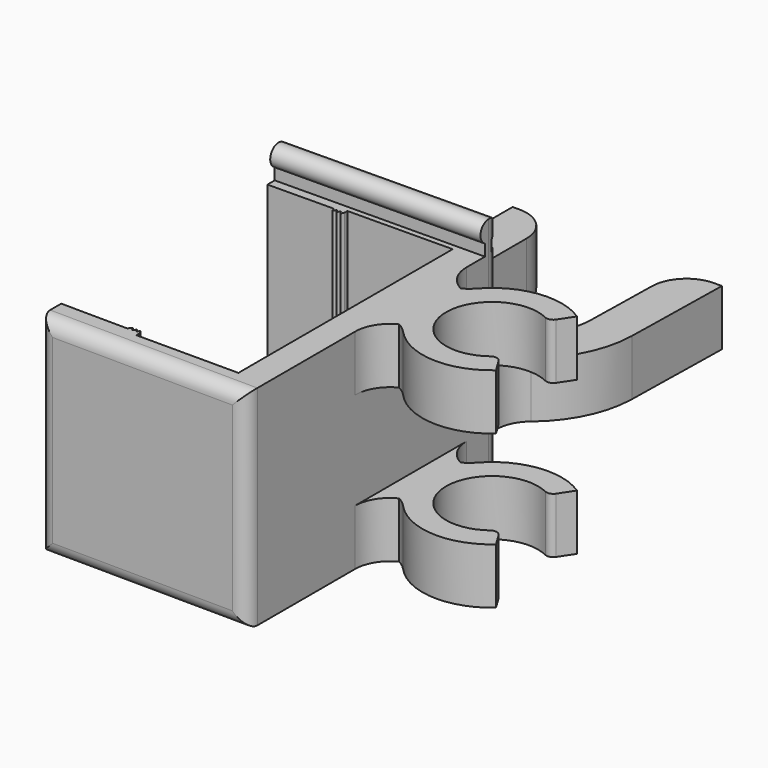
from build123d import *

# Parameters (mm, degrees)
F1_DEPTH     = 30
F2_DEPTH     = 8
F5_DEPTH     = 8
F6_W         = 15
F6_H         = 8
F7_DEPTH     = 17
F10_DEPTH    = 8
F12_REACH    = 53.956775782
F13_T1_DEPTH = 8
F13_T3_DEPTH = 8
F13_T5_DEPTH = 33
F13_T7_DEPTH = 32.520696372
F14_R        = 2
F15_R        = 1


# Not quite as in the source:
# - a fillet or chamfer that OpenCascade refuses, or shapes differently, is made with other operations: its cross-section is extruded or revolved along the edge and cut away or added


with BuildPart() as f1:
    # F0 (on Top) → F1 (new body)
    with BuildSketch(Plane.XY):
        Polygon((-19.4335049985, 21.8533294287), (-19.3985988565, 17.8534817365), (-9.9558601587, 17.9358872687), (-9.7491024062, 17.4549428523), (-9.4364569921, 17.9404200315), (-9.1781169176, 17.4304714203), (-8.9225616318, 17.9449047283), (-8.6024082196, 17.4476796256), (-8.3908626536, 17.949544795), (-8.3952257552, 18.4495067188), (6.6091373464, 18.5804478119), (6.6091373464, 18.0804478119), (6.6091373464, -19.3734843389), (6.6259289407, -19.8732023017), (-8.0640320303, -19.8732023017), (-8.0233838527, -19.2457882609), (-8.3196364677, -18.7431838643), (-8.5862603211, -19.2408761124), (-8.8343713433, -18.7508519739), (-9.1803468433, -19.2356915979), (-9.4099212438, -18.7637861818), (-9.9014025182, -19.2293990403), (-19.3985988565, -19.1465182635), (-19.3985988565, -23.1465182635), (10.5653526934, -23.4080097072), (10.5653526934, 1.1284245411), (10.5653526934, 11.1284245411), (10.5653526934, 22.1151254937), align=None)
    extrude(amount=F1_DEPTH)

    # F0 (on Top) → F2 (join)
    with BuildSketch(Plane.XY):
        with BuildLine():
            Line((13.4887376895, 11.1284245411), (10.5653526934, 11.1284245411))
            Line((10.5653526934, 11.1284245411), (10.5653526934, 1.1284245411))
            Line((10.5653526934, 1.1284245411), (13.558922693, 1.1284245411))
            ThreePointArc((13.558922693, 1.1284245411), (20.5784668777, -3.6810997137), (28.7603608072, -1.3439784408))
            Line((28.7603608072, -1.3439784408), (27.5756506747, 0.610225606))
            ThreePointArc((27.5756506747, 0.610225606), (26.9123854989, 1.0732349365), (26.1235827728, 0.8941020455))
            ThreePointArc((26.1235827728, 0.8941020455), (15.6131288756, 5.5676877801), (25.0608685177, 12.1291099125))
            ThreePointArc((25.0608685177, 12.1291099125), (25.7618549762, 12.0648655681), (26.3314982765, 12.4784062083))
            Line((26.3314982765, 12.4784062083), (27.6896333508, 14.5370064881))
            ThreePointArc((27.6896333508, 14.5370064881), (19.8498327125, 15.9130205333), (13.4887376895, 11.1284245411))
        make_face()
    extrude(amount=F2_DEPTH)

    # F4 (on offset) → F5 (join, through all)
    with BuildSketch(Plane.XY.offset(22)):
        with BuildLine():
            Line((13.4887376895, 11.1284245411), (10.5653526934, 11.1284245411))
            Line((10.5653526934, 11.1284245411), (10.5653526934, 1.1284245411))
            Line((10.5653526934, 1.1284245411), (13.558922693, 1.1284245411))
            ThreePointArc((13.558922693, 1.1284245411), (20.5784668777, -3.6810997137), (28.7603608072, -1.3439784408))
            Line((28.7603608072, -1.3439784408), (27.5756506747, 0.610225606))
            ThreePointArc((27.5756506747, 0.610225606), (26.9123854989, 1.0732349365), (26.1235827728, 0.8941020455))
            ThreePointArc((26.1235827728, 0.8941020455), (15.6131288756, 5.5676877801), (25.0608685177, 12.1291099125))
            ThreePointArc((25.0608685177, 12.1291099125), (25.7618549762, 12.0648655681), (26.3314982765, 12.4784062083))
            Line((26.3314982765, 12.4784062083), (27.6896333508, 14.5370064881))
            ThreePointArc((27.6896333508, 14.5370064881), (19.8498327125, 15.9130205333), (13.4887376895, 11.1284245411))
        make_face()
    extrude(amount=F5_DEPTH)

    # F6 (on face) → F7 (join)
    with BuildSketch(Plane(origin=(-0.1921765021, 22.0212459587, 0), x_dir=(-0.9999619231, -0.0087265355, 0), z_dir=(-0.0087265355, 0.9999619231, 0))):
        with Locations((5.4527436662, 4)):
            Rectangle(F6_W, F6_H)
    extrude(amount=F7_DEPTH)

    # F9 (on offset) → F10 (join, through all)
    with BuildSketch(Plane.XY.offset(8)):
        with BuildLine():
            ThreePointArc((-5.8678184254, 38.9723627145), (-12.3220017893, 41.6197640951), (-14.945665031, 48.0836335368))
            Line((-14.945665031, 48.0836335368), (-14.945665031, 63.7743831428))
            Line((-14.945665031, 63.7743831428), (-20.9462765716, 63.7743831428))
            Line((-20.9462765716, 63.7743831428), (-20.9462765716, 48.0211850887))
            ThreePointArc((-20.9462765716, 48.0211850887), (-6.1161143863, 32.9729806378), (9.0508327111, 47.681681579))
            Line((9.0508327111, 47.681681579), (9.3561656724, 63.4534007051))
            Line((9.3561656724, 63.4534007051), (3.3550414043, 63.4534007051))
            Line((3.3550414043, 63.4534007051), (3.0519567686, 47.7978169566))
            ThreePointArc((3.0519567686, 47.7978169566), (0.3836882004, 41.5743230997), (-5.8678184254, 38.9723627145))
        make_face()
    extrude(amount=-F10_DEPTH)

    f12_end = Plane(origin=(10.5653526934, -1.5454916278, 15), x_dir=(0, 1, 0), z_dir=(1, 0, 0))
    # F11 (on face) → F12 (join, up to a plane its end follows)
    with BuildSketch(Plane(origin=(-19.2413284964, -0.1679165299, 0), x_dir=(0.0087265355, -0.9999619231, 0), z_dir=(-0.9999619231, -0.0087265355, 0))):
        with BuildLine():
            Line((-20.7125834072, 30), (-19.3315855771, 30))
            Line((-19.3315855771, 30), (-19.3315855771, 31.6558666838))
            ThreePointArc((-19.3315855771, 31.6558666838), (-20.0220844921, 34.4874864675), (-20.7125834072, 31.6558666838))
            Line((-20.7125834072, 31.6558666838), (-20.7125834072, 30))
        make_face()
    f12_long = extrude(amount=-F12_REACH, mode=Mode.PRIVATE)
    add(split(f12_long, bisect_by=f12_end, keep=Keep.BOTTOM, mode=Mode.PRIVATE))

    # F13: fillet of radius 5 on 14 edges, made by hand

    # F13_s2 → F13_t1 (join)
    with BuildSketch(Plane.XY):
        with BuildLine():
            ThreePointArc((-18.1442365828, 21.8645807038), (-14.6216170146, 23.3598439976), (-13.188059645, 26.9080229966))
            Line((-13.188059645, 26.9080229966), (-13.1444269675, 21.9082133812))
            Line((-13.1444269675, 21.9082133812), (-18.1442365828, 21.8645807038))
        make_face()
        with BuildLine():
            ThreePointArc((6.8548114938, 22.0827440912), (3.3066324948, 23.5163014608), (1.8113692009, 27.038921029))
            Line((1.8113692009, 27.038921029), (1.8550018784, 22.0391114137))
            Line((1.8550018784, 22.0391114137), (6.8548114938, 22.0827440912))
        make_face()
        with BuildLine():
            ThreePointArc((10.5653526934, 16.1284245411), (12.0298187875, 12.5928906352), (15.5653526934, 11.1284245411))
            Line((15.5653526934, 11.1284245411), (10.5653526934, 11.1284245411))
            Line((10.5653526934, 11.1284245411), (10.5653526934, 16.1284245411))
        make_face()
        with BuildLine():
            ThreePointArc((10.5653526934, -3.8715754589), (12.0298187875, -0.336041553), (15.5653526934, 1.1284245411))
            Line((15.5653526934, 1.1284245411), (10.5653526934, 1.1284245411))
            Line((10.5653526934, 1.1284245411), (10.5653526934, -3.8715754589))
        make_face()
        with BuildLine():
            ThreePointArc((11.0581220717, 1.1284245411), (13.0869189237, 0.6983242482), (14.7666813277, -0.5179821256))
            ThreePointArc((14.7666813277, -0.5179821256), (14.12066956, 0.2743140014), (13.558922693, 1.1284245411))
            Line((13.558922693, 1.1284245411), (11.0581220717, 1.1284245411))
        make_face()
        with BuildLine():
            ThreePointArc((14.69419502, 12.8153512078), (13.0030032517, 11.5696217012), (10.9493926103, 11.1284245411))
            Line((10.9493926103, 11.1284245411), (13.4887376895, 11.1284245411))
            ThreePointArc((13.4887376895, 11.1284245411), (14.0476280356, 12.0032142055), (14.69419502, 12.8153512078))
        make_face()
        with BuildLine():
            ThreePointArc((1.7638300569, 32.4863673707), (2.2328927557, 34.644789016), (3.5861404679, 36.3905050419))
            ThreePointArc((3.5861404679, 36.3905050419), (2.6880734851, 35.7063521777), (1.7410938173, 35.0916823838))
            Line((1.7410938173, 35.0916823838), (1.7638300569, 32.4863673707))
        make_face()
        with BuildLine():
            ThreePointArc((-13.2345541346, 32.2357638009), (-13.7517699867, 34.4071600518), (-15.1623620988, 36.1371033483))
            ThreePointArc((-15.1623620988, 36.1371033483), (-14.2340524811, 35.4694560451), (-13.2575817153, 34.8744631788))
            Line((-13.2575817153, 34.8744631788), (-13.2345541346, 32.2357638009))
        make_face()
    extrude(amount=F13_T1_DEPTH)

    # F13_s4 → F13_t3 (join)
    with BuildSketch(Plane.XY.offset(22)):
        with BuildLine():
            ThreePointArc((10.5653526934, 16.1284245411), (12.0298187875, 12.5928906352), (15.5653526934, 11.1284245411))
            Line((15.5653526934, 11.1284245411), (10.5653526934, 11.1284245411))
            Line((10.5653526934, 11.1284245411), (10.5653526934, 16.1284245411))
        make_face()
        with BuildLine():
            ThreePointArc((10.5653526934, -3.8715754589), (12.0298187875, -0.336041553), (15.5653526934, 1.1284245411))
            Line((15.5653526934, 1.1284245411), (10.5653526934, 1.1284245411))
            Line((10.5653526934, 1.1284245411), (10.5653526934, -3.8715754589))
        make_face()
        with BuildLine():
            ThreePointArc((10.9493926103, 11.1284245411), (13.0030032517, 11.5696217012), (14.69419502, 12.8153512078))
            ThreePointArc((14.69419502, 12.8153512078), (14.0476280356, 12.0032142055), (13.4887376895, 11.1284245411))
            Line((13.4887376895, 11.1284245411), (10.9493926103, 11.1284245411))
        make_face()
        with BuildLine():
            ThreePointArc((11.0581220717, 1.1284245411), (13.0869189237, 0.6983242482), (14.7666813277, -0.5179821256))
            ThreePointArc((14.7666813277, -0.5179821256), (14.12066956, 0.2743140014), (13.558922693, 1.1284245411))
            Line((13.558922693, 1.1284245411), (11.0581220717, 1.1284245411))
        make_face()
    extrude(amount=F13_T3_DEPTH)

    # F13_s6 → F13_t5 (cut)
    with BuildSketch(Plane.XY.offset(-12.5)):
        with BuildLine():
            ThreePointArc((-14.945665031, 58.7743831428), (-16.4101311251, 62.3099170488), (-19.945665031, 63.7743831428))
            Line((-19.945665031, 63.7743831428), (-14.945665031, 63.7743831428))
            Line((-14.945665031, 63.7743831428), (-14.945665031, 58.7743831428))
        make_face()
    extrude(amount=F13_T5_DEPTH, mode=Mode.SUBTRACT)

    # F13_s8 → F13_t7 (cut)
    with BuildSketch(Plane.XY.offset(-12.260348186)):
        with BuildLine():
            ThreePointArc((8.2591806787, 63.4534007051), (4.7580306824, 62.0229873343), (3.2601173933, 58.5501801864))
            Line((3.2601173933, 58.5501801864), (3.3550414043, 63.4534007051))
            Line((3.3550414043, 63.4534007051), (8.2591806787, 63.4534007051))
        make_face()
    extrude(amount=F13_T7_DEPTH, mode=Mode.SUBTRACT)

    # F14
    f14_edges = [f1.edges().sort_by_distance(p)[0] for p in [
        (10.565353, -23.40801, 15),
        (-4.416623, -23.277264, 30),
        (-19.398599, -23.146518, 15),
        (-4.416623, -23.277264, 0),
        (10.565353, 22.115125, 15),
    ]]
    fillet(f14_edges, radius=F14_R)

    # F15
    f15_edges = [f1.edges().sort_by_distance(p)[0] for p in [
        (-19.433505, 21.853329, 15),
    ]]
    fillet(f15_edges, radius=F15_R)


solid = f1.part
